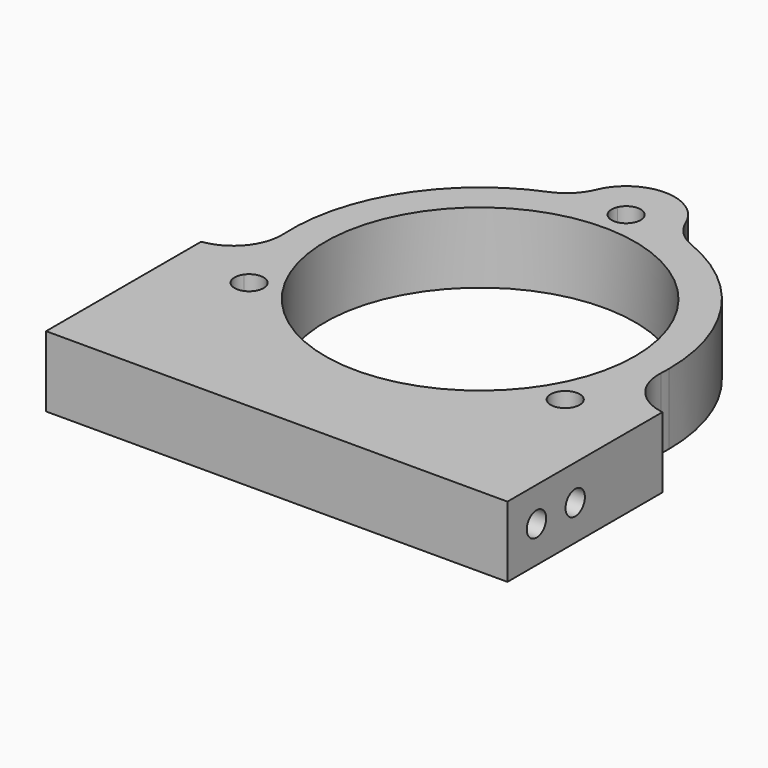
from build123d import *

# Parameters (mm, degrees)
F0_R     = 20.32
F1_DEPTH = 9.271
F2_R     = 1.5875
F3_DEPTH = 60.511199891
F4_R     = 6.35


# Not quite as in the source:
# - a feature names something its author has since deleted; it is built from what else it names


with BuildPart() as f1:
    # F0 (on Top) → F1 (new body)
    with BuildSketch(Plane.XY):
        with BuildLine():
            ThreePointArc((23.9050999455, -6.4692674698), (24.5490837421, -3.2630832697), (24.765, 0))
            ThreePointArc((24.765, 0), (19.6285885254, 15.1004548773), (6.35, 23.9370575677))
            ThreePointArc((6.35, 23.9370575677), (4.0651088886, 24.4290833787), (1.7440091422, 24.703515076))
            ThreePointArc((1.7440091422, 24.703515076), (1.8643178935, 24.3286489263), (1.905, 23.9370575677))
            ThreePointArc((1.905, 23.9370575677), (-0.3915913586, 22.0727396742), (-1.7440091422, 24.703515076))
            ThreePointArc((-1.7440091422, 24.703515076), (-4.0651088886, 24.4290833787), (-6.35, 23.9370575677))
            ThreePointArc((-6.35, 23.9370575677), (-21.4471191247, 12.3825), (-23.9050999455, -6.4692674698))
            ThreePointArc((-23.9050999455, -6.4692674698), (-23.1887612414, -8.6940541227), (-22.2658761897, -10.8414013165))
            ThreePointArc((-22.2658761897, -10.8414013165), (-20.1370690632, -10.1581864481), (-18.8250999455, -11.9685287839))
            ThreePointArc((-18.8250999455, -11.9685287839), (-19.3113489683, -13.239815795), (-20.5218670475, -13.8621137596))
            ThreePointArc((-20.5218670475, -13.8621137596), (-19.1236523528, -15.735029256), (-17.5550999455, -17.4677900979))
            ThreePointArc((-17.5550999455, -17.4677900979), (0, -24.765), (17.5550999455, -17.4677900979))
            ThreePointArc((17.5550999455, -17.4677900979), (19.1236523528, -15.735029256), (20.5218670475, -13.8621137596))
            ThreePointArc((20.5218670475, -13.8621137596), (19.0803215513, -11.0160287839), (22.2658761897, -10.8414013165))
            ThreePointArc((22.2658761897, -10.8414013165), (23.1887612414, -8.6940541227), (23.9050999455, -6.4692674698))
        make_face()
        Circle(F0_R, mode=Mode.SUBTRACT)
        with BuildLine():
            ThreePointArc((-22.2658761897, -10.8414013165), (-23.1887612414, -8.6940541227), (-23.9050999455, -6.4692674698))
            ThreePointArc((-23.9050999455, -6.4692674698), (-26.2293612595, -15.1435287839), (-17.5550999455, -17.4677900979))
            ThreePointArc((-17.5550999455, -17.4677900979), (-19.1236523528, -15.735029256), (-20.5218670475, -13.8621137596))
            ThreePointArc((-20.5218670475, -13.8621137596), (-22.3798783397, -12.9210287839), (-22.2658761897, -10.8414013165))
        make_face()
        with BuildLine():
            ThreePointArc((17.5550999455, -17.4677900979), (26.2293612595, -15.1435287839), (23.9050999455, -6.4692674698))
            ThreePointArc((23.9050999455, -6.4692674698), (23.1887612414, -8.6940541227), (22.2658761897, -10.8414013165))
            ThreePointArc((22.2658761897, -10.8414013165), (22.5404422812, -11.3754979015), (22.6350999455, -11.9685287839))
            ThreePointArc((22.6350999455, -11.9685287839), (22.0013869566, -13.3872797611), (20.5218670475, -13.8621137596))
            ThreePointArc((20.5218670475, -13.8621137596), (19.1236523528, -15.735029256), (17.5550999455, -17.4677900979))
        make_face()
        with BuildLine():
            Line((30.2550999455, -7.9427900979), (23.9050999455, -6.4692674698))
            ThreePointArc((23.9050999455, -6.4692674698), (26.2293612595, -15.1435287839), (17.5550999455, -17.4677900979))
            ThreePointArc((17.5550999455, -17.4677900979), (0, -24.765), (-17.5550999455, -17.4677900979))
            ThreePointArc((-17.5550999455, -17.4677900979), (-26.2293612595, -15.1435287839), (-23.9050999455, -6.4692674698))
            Line((-23.9050999455, -6.4692674698), (-30.2550999455, -7.9427900979))
            Line((-30.2550999455, -7.9427900979), (-30.2550999455, -33.3427900979))
            Line((-30.2550999455, -33.3427900979), (30.2550999455, -33.3427900979))
            Line((30.2550999455, -33.3427900979), (30.2550999455, -7.9427900979))
        make_face()
        with BuildLine():
            ThreePointArc((1.7440091422, 24.703515076), (4.0651088886, 24.4290833787), (6.35, 23.9370575677))
            ThreePointArc((6.35, 23.9370575677), (0, 30.2870575677), (-6.35, 23.9370575677))
            ThreePointArc((-6.35, 23.9370575677), (-4.0651088886, 24.4290833787), (-1.7440091422, 24.703515076))
            ThreePointArc((-1.7440091422, 24.703515076), (0, 25.8420575677), (1.7440091422, 24.703515076))
        make_face()
    extrude(amount=F1_DEPTH)

    # F2 (on face) → F3 (cut, through all)
    with BuildSketch(Plane.YZ.offset(30.2550999455)):
        with Locations((-28.5802900979, 4.7625)):
            Circle(F2_R)
        with Locations((-22.2315602249, 4.6355)):
            Circle(F2_R)
    extrude(amount=-F3_DEPTH, mode=Mode.SUBTRACT)

    # F4
    f4_edges = [f1.edges().sort_by_distance(p)[0] for p in [
        (-23.9051, -6.469267, 4.6355),
        (23.9051, -6.469267, 4.6355),
        (6.35, 23.937058, 4.6355),
        (-6.35, 23.937058, 4.6355),
    ]]
    fillet(f4_edges, radius=F4_R)


solid = f1.part
